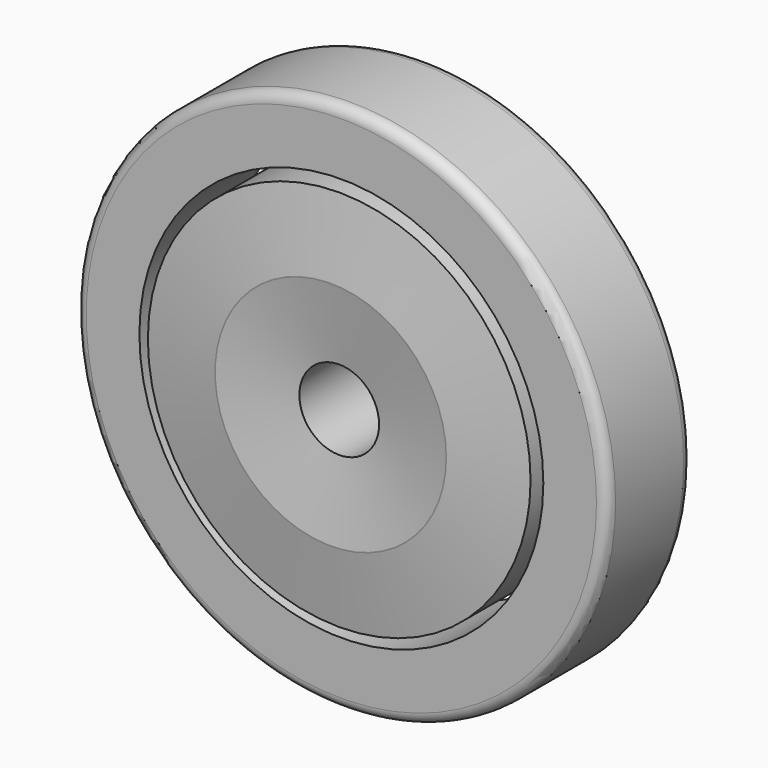
from build123d import *

# Parameters (mm, degrees)
F0_R        = 63.5
F0_R_2      = 48.26
F1_DEPTH    = 12.7
F2_R        = 2.54
F3_R        = 45.72
F3_R_2      = 9.525
F4_DEPTH    = 15.875
F5_C1_SIZE2 = 18.034
F5_C1_SIZE  = 2.54
F5_C2_SIZE2 = 2.54
F5_C2_SIZE  = 18.034
F6_SIZE2    = 17.78
F6_SIZE     = 2.54


with BuildPart() as f1:
    # F0 (on Front) → F1 (new body, symmetric)
    with BuildSketch(Plane.XZ):
        Circle(F0_R)
        Circle(F0_R_2, mode=Mode.SUBTRACT)
    extrude(amount=F1_DEPTH, both=True)

    # F2
    f2_edges = [f1.edges().sort_by_distance(p)[0] for p in [
        (-63.5, 12.7, 0),
        (63.5, 0, 0),
        (-63.5, -12.7, 0),
    ]]
    fillet(f2_edges, radius=F2_R)


with BuildPart() as f4:
    # F3 (on Front) → F4 (new body, symmetric)
    with BuildSketch(Plane.XZ):
        Circle(F3_R)
        Circle(F3_R_2, mode=Mode.SUBTRACT)
    extrude(amount=F4_DEPTH, both=True)

    # F5: chamfer of 18.034 x 2.54 on 2 edges, made by hand

    # F5_c1
    f5_c1_edges = [f4.edges().sort_by_distance(p)[0] for p in [
        (-45.72, -15.875, 0),
    ]]
    f5_c1_side = f4.faces().sort_by_distance((-45.72, -15.8242, 0))[0]
    chamfer(f5_c1_edges, length=F5_C1_SIZE, length2=F5_C1_SIZE2, reference=f5_c1_side)

    # F5_c2
    f5_c2_edges = [f4.edges().sort_by_distance(p)[0] for p in [
        (-9.525, -15.875, 0),
    ]]
    f5_c2_side = f4.faces().sort_by_distance((-9.5758, -15.875, 0))[0]
    chamfer(f5_c2_edges, length=F5_C2_SIZE, length2=F5_C2_SIZE2, reference=f5_c2_side)

    # F6
    f6_edges = [f4.edges().sort_by_distance(p)[0] for p in [
        (-45.72, 15.875, 0),
        (-9.525, 15.875, 0),
    ]]
    chamfer(f6_edges, length=F6_SIZE, length2=F6_SIZE2)


solid = Compound([f1.part, f4.part])
